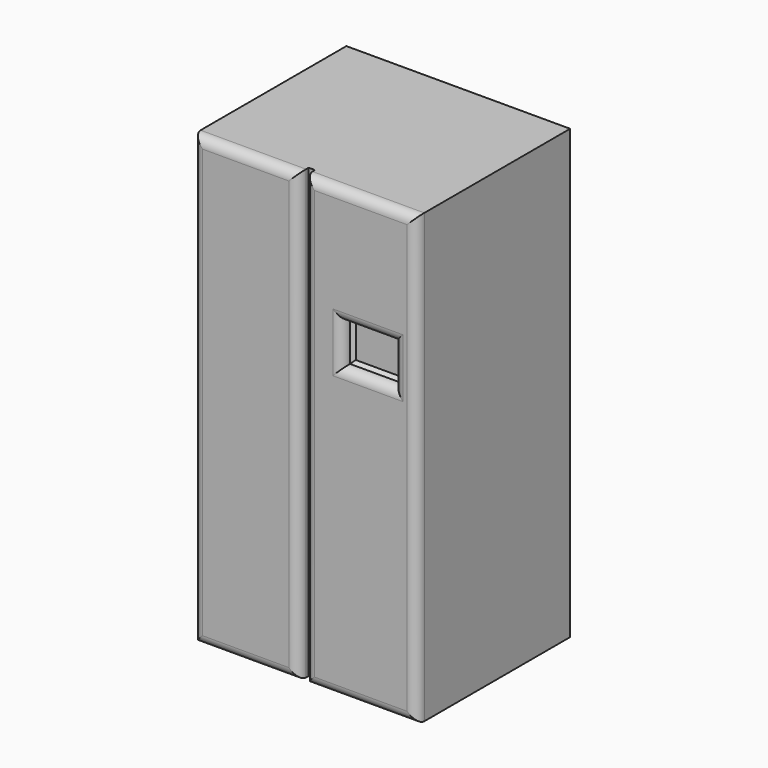
from build123d import *

# Parameters (mm, degrees)
F0_W     = 889
F0_H     = 762
F1_DEPTH = 1778
F2_W     = 25.4
F2_H     = 1778
F3_DEPTH = 50.8
F4_W     = 203.0948400497
F4_H     = 157.5736999512
F5_DEPTH = 50.8
F6_SIZE  = 12.7
F7_R     = 38.09999


# Not quite as in the source:
# - a fillet or chamfer is up to 0.001 mm smaller than in the source, because OpenCascade refuses the exact size


with BuildPart() as f1:
    # F0 (on Top) → F1 (new body)
    with BuildSketch(Plane.XY):
        with Locations((444.5, 381)):
            Rectangle(F0_W, F0_H)
    extrude(amount=F1_DEPTH)

    # F2 (on face) → F3 (cut)
    with BuildSketch(Plane.XZ):
        with Locations((431.8, 889)):
            Rectangle(F2_W, F2_H)
    extrude(amount=-F3_DEPTH, mode=Mode.SUBTRACT)

    # F4 (on face) → F5 (cut)
    with BuildSketch(Plane.XZ):
        with Locations((695.2850222588, 1232.5783967972)):
            Rectangle(F4_W, F4_H)
    extrude(amount=-F5_DEPTH, mode=Mode.SUBTRACT)

    # F6
    f6_edges = [f1.edges().sort_by_distance(p)[0] for p in [
        (695.285022, 50.8, 1311.365247),
        (593.737602, 50.8, 1232.578397),
        (695.285022, 50.8, 1153.791547),
        (796.832442, 50.8, 1232.578397),
    ]]
    chamfer(f6_edges, length=F6_SIZE)

    # F7 (radius 38.1 in the source; OpenCascade refuses exactly that, so slightly less here)
    f7_edges = [f1.edges().sort_by_distance(p)[0] for p in [
        (209.55, 0, 0),
        (419.1, 0, 889),
        (209.55, 0, 1778),
        (0, 0, 889),
        (666.75, 0, 0),
        (444.5, 0, 889),
        (889, 0, 889),
        (666.75, 0, 1778),
        (796.832442, 0, 1232.578397),
        (695.285022, 0, 1153.791547),
        (593.737602, 0, 1232.578397),
        (695.285022, 0, 1311.365247),
    ]]
    fillet(f7_edges, radius=F7_R)


solid = f1.part
